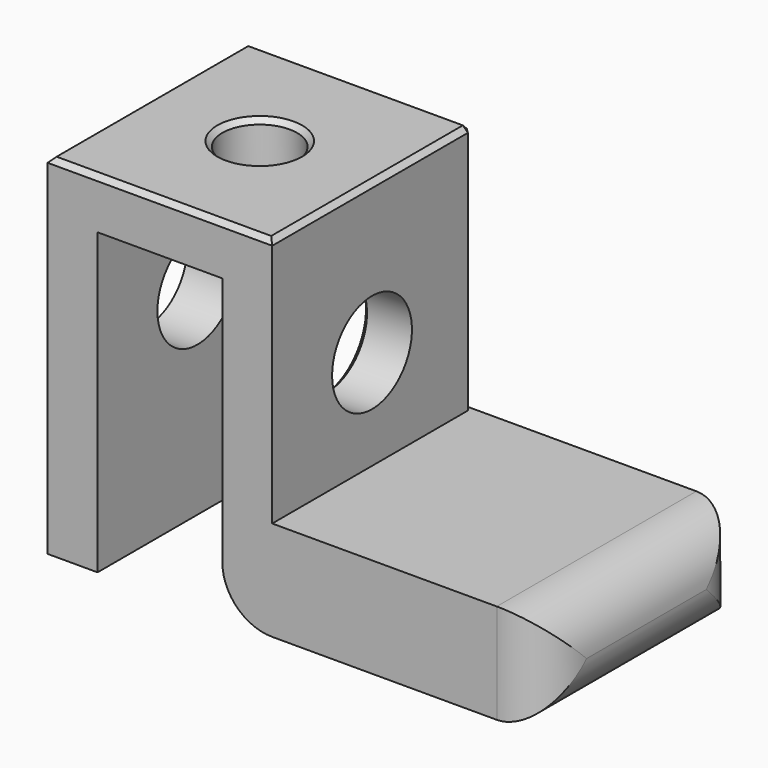
from build123d import *

# Parameters (mm, degrees)
F0_W     = 100
F0_H     = 50
F1_DEPTH = 20
F2_W     = 45
F2_H     = 50
F3_DEPTH = 50
F4_W     = 25
F4_H     = 60
F5_DEPTH = 50.001
F6_R     = 10
F7_DEPTH = 45
F8_R     = 7.5
F9_DEPTH = 70.001
F10_SIZE = 1
F11_R    = 9.99999


# Not quite as in the source:
# - a fillet or chamfer is up to 0.001 mm smaller than in the source, because OpenCascade refuses the exact size


with BuildPart() as f1:
    # F0 (on Top) → F1 (new body)
    with BuildSketch(Plane.XY):
        with Locations((50, 25)):
            Rectangle(F0_W, F0_H)
    extrude(amount=F1_DEPTH)

    # F2 (on face) → F3 (join)
    with BuildSketch(Plane.XY.offset(20)):
        with Locations((22.5, 25)):
            Rectangle(F2_W, F2_H)
    extrude(amount=F3_DEPTH)

    # F4 (on face) → F5 (cut, through all)
    with BuildSketch(Plane.XZ):
        with Locations((22.5, 30)):
            Rectangle(F4_W, F4_H)
    extrude(amount=-F5_DEPTH, mode=Mode.SUBTRACT)

    # F6 (on face) → F7 (cut, through all)
    with BuildSketch(Plane(origin=(0, 0, 0), x_dir=(0, -1, 0), z_dir=(-1, 0, 0))):
        with Locations((-25, 40)):
            Circle(F6_R)
    extrude(amount=-F7_DEPTH, mode=Mode.SUBTRACT)

    # F8 (on face) → F9 (cut, through all)
    with BuildSketch(Plane.XY.offset(70)):
        with Locations((22.5, 25)):
            Circle(F8_R)
    extrude(amount=-F9_DEPTH, mode=Mode.SUBTRACT)

    # F10
    f10_edges = [f1.edges().sort_by_distance(p)[0] for p in [
        (45, 50, 45),
        (22.5, 50, 70),
        (45, 25, 70),
        (0, 25, 70),
        (0, 50, 35),
        (10, 50, 30),
        (22.5, 50, 60),
        (35, 50, 30),
        (35, 35, 40),
        (15, 25, 70),
        (22.5, 0, 70),
    ]]
    chamfer(f10_edges, length=F10_SIZE)

    # F11 (radius 10 in the source; OpenCascade refuses exactly that, so slightly less here)
    f11_edges = [f1.edges().sort_by_distance(p)[0] for p in [
        (35, 24.5, 0),
        (100, 25, 0),
        (100, 0, 10),
        (100, 25, 20),
        (100, 50, 10),
    ]]
    fillet(f11_edges, radius=F11_R)


solid = f1.part
